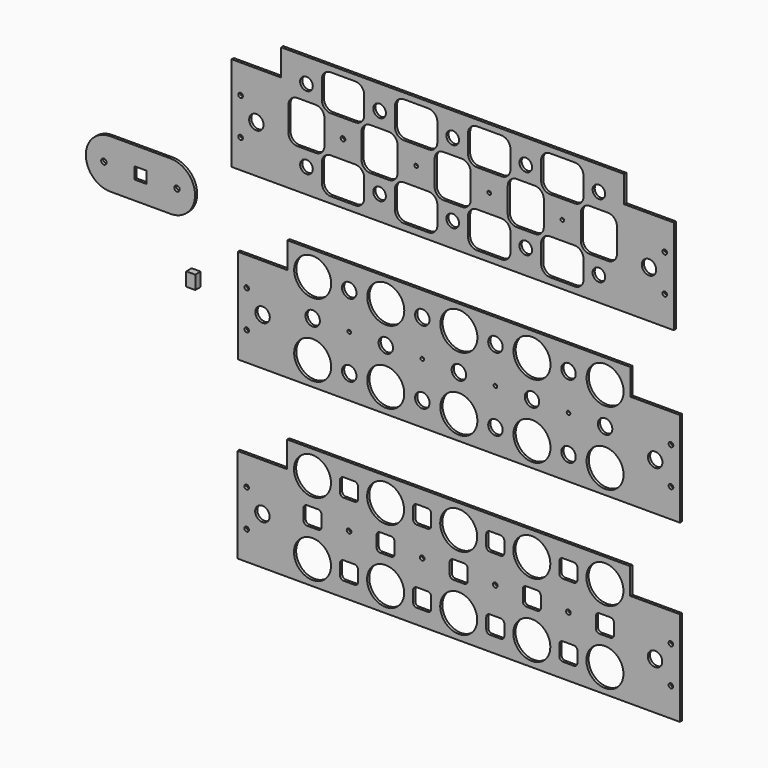
from build123d import *

# Parameters (mm, degrees)
F0_R     = 2.55
F0_R_2   = 8
F0_R_3   = 7
F0_R_4   = 2
F1_DEPTH = 3
F0_R_5   = 20.5
F0_W     = 20
F0_H     = 20
F2_DEPTH = 3
F0_R_6   = 3
F0_W_2   = 13
F0_H_2   = 13
F0_W_3   = 10
F0_H_3   = 15
F3_DEPTH = 4.5


# Not quite as in the source:
# - a feature names something its author has since deleted; it is built from what else it names


with BuildPart() as f1:
    # F0 (on Front) → F1 (new body)
    with BuildSketch(Plane.XZ):
        Polygon((-471.3846094865, 146.640773439), (-471.3846094865, 251.640773439), (-506.3846094865, 251.640773439), (-506.3846094865, 231.640773439), (-526.3846094865, 231.640773439), (-526.3846094865, 166.640773439), (-506.3846094865, 166.640773439), (-506.3846094865, 146.640773439), align=None)
        with Locations((-516.3846094865, 178.640773439)):
            Circle(F0_R, mode=Mode.SUBTRACT)
        with Locations((-498.8846094865, 199.140773439)):
            Circle(F0_R_2, mode=Mode.SUBTRACT)
        with Locations((-516.3846094865, 219.640773439)):
            Circle(F0_R, mode=Mode.SUBTRACT)
        Polygon((-56.3846094865, 251.640773439), (-91.3846094865, 251.640773439), (-91.3846094865, 146.640773439), (-56.3846094865, 146.640773439), (-56.3846094865, 166.640773439), (-36.3846094865, 166.640773439), (-36.3846094865, 231.640773439), (-56.3846094865, 231.640773439), align=None)
        with Locations((-46.3846094865, 178.640773439)):
            Circle(F0_R, mode=Mode.SUBTRACT)
        with Locations((-63.8846094865, 199.140773439)):
            Circle(F0_R_2, mode=Mode.SUBTRACT)
        with Locations((-46.3846094865, 219.640773439)):
            Circle(F0_R, mode=Mode.SUBTRACT)
        Polygon((-91.3846094865, 281.140773439), (-471.3846094865, 281.140773439), (-471.3846094865, 251.640773439), (-471.3846094865, 146.640773439), (-91.3846094865, 146.640773439), (-91.3846094865, 251.640773439), align=None)
        with Locations((-443.3846094865, 173.640773439)):
            Circle(F0_R_3, mode=Mode.SUBTRACT)
        with BuildLine():
            ThreePointArc((-433.399160381, 237.5500709947), (-426.3280925692, 234.6211388066), (-423.399160381, 227.5500709947))
            Line((-423.399160381, 227.5500709947), (-423.399160381, 200.5500709947))
            ThreePointArc((-423.399160381, 200.5500709947), (-426.3280925692, 193.4790031828), (-433.399160381, 190.5500709947))
            Line((-433.399160381, 190.5500709947), (-453.399160381, 190.5500709947))
            ThreePointArc((-453.399160381, 190.5500709947), (-460.4702281929, 193.4790031828), (-463.399160381, 200.5500709947))
            Line((-463.399160381, 200.5500709947), (-463.399160381, 227.5500709947))
            ThreePointArc((-463.399160381, 227.5500709947), (-460.4702281929, 234.6211388066), (-453.399160381, 237.5500709947))
            Line((-453.399160381, 237.5500709947), (-433.399160381, 237.5500709947))
        make_face(mode=Mode.SUBTRACT)
        with BuildLine():
            ThreePointArc((-379.3846094865, 163.640773439), (-382.3135416747, 156.5697056271), (-389.3846094865, 153.640773439))
            Line((-389.3846094865, 153.640773439), (-416.3846094865, 153.640773439))
            ThreePointArc((-416.3846094865, 153.640773439), (-423.4556772984, 156.5697056271), (-426.3846094865, 163.640773439))
            Line((-426.3846094865, 163.640773439), (-426.3846094865, 183.640773439))
            ThreePointArc((-426.3846094865, 183.640773439), (-423.4556772984, 190.7118412509), (-416.3846094865, 193.640773439))
            Line((-416.3846094865, 193.640773439), (-389.3846094865, 193.640773439))
            ThreePointArc((-389.3846094865, 193.640773439), (-382.3135416747, 190.7118412509), (-379.3846094865, 183.640773439))
            Line((-379.3846094865, 183.640773439), (-379.3846094865, 163.640773439))
        make_face(mode=Mode.SUBTRACT)
        with Locations((-362.3846094865, 173.640773439)):
            Circle(F0_R_3, mode=Mode.SUBTRACT)
        with Locations((-402.8846094865, 214.140773439)):
            Circle(F0_R, mode=Mode.SUBTRACT)
        with BuildLine():
            ThreePointArc((-352.399160381, 237.5500709947), (-345.3280925692, 234.6211388066), (-342.399160381, 227.5500709947))
            Line((-342.399160381, 227.5500709947), (-342.399160381, 200.5500709947))
            ThreePointArc((-342.399160381, 200.5500709947), (-345.3280925692, 193.4790031828), (-352.399160381, 190.5500709947))
            Line((-352.399160381, 190.5500709947), (-372.399160381, 190.5500709947))
            ThreePointArc((-372.399160381, 190.5500709947), (-379.4702281929, 193.4790031828), (-382.399160381, 200.5500709947))
            Line((-382.399160381, 200.5500709947), (-382.399160381, 227.5500709947))
            ThreePointArc((-382.399160381, 227.5500709947), (-379.4702281929, 234.6211388066), (-372.399160381, 237.5500709947))
            Line((-372.399160381, 237.5500709947), (-352.399160381, 237.5500709947))
        make_face(mode=Mode.SUBTRACT)
        with Locations((-443.3846094865, 254.640773439)):
            Circle(F0_R_3, mode=Mode.SUBTRACT)
        with BuildLine():
            ThreePointArc((-379.3846094865, 244.640773439), (-382.3135416747, 237.5697056271), (-389.3846094865, 234.640773439))
            Line((-389.3846094865, 234.640773439), (-416.3846094865, 234.640773439))
            ThreePointArc((-416.3846094865, 234.640773439), (-423.4556772984, 237.5697056271), (-426.3846094865, 244.640773439))
            Line((-426.3846094865, 244.640773439), (-426.3846094865, 264.640773439))
            ThreePointArc((-426.3846094865, 264.640773439), (-423.4556772984, 271.7118412509), (-416.3846094865, 274.640773439))
            Line((-416.3846094865, 274.640773439), (-389.3846094865, 274.640773439))
            ThreePointArc((-389.3846094865, 274.640773439), (-382.3135416747, 271.7118412509), (-379.3846094865, 264.640773439))
            Line((-379.3846094865, 264.640773439), (-379.3846094865, 244.640773439))
        make_face(mode=Mode.SUBTRACT)
        with Locations((-362.3846094865, 254.640773439)):
            Circle(F0_R_3, mode=Mode.SUBTRACT)
        with BuildLine():
            ThreePointArc((-298.3846094865, 163.640773439), (-301.3135416747, 156.5697056271), (-308.3846094865, 153.640773439))
            Line((-308.3846094865, 153.640773439), (-335.3846094865, 153.640773439))
            ThreePointArc((-335.3846094865, 153.640773439), (-342.4556772984, 156.5697056271), (-345.3846094865, 163.640773439))
            Line((-345.3846094865, 163.640773439), (-345.3846094865, 183.640773439))
            ThreePointArc((-345.3846094865, 183.640773439), (-342.4556772984, 190.7118412509), (-335.3846094865, 193.640773439))
            Line((-335.3846094865, 193.640773439), (-308.3846094865, 193.640773439))
            ThreePointArc((-308.3846094865, 193.640773439), (-301.3135416747, 190.7118412509), (-298.3846094865, 183.640773439))
            Line((-298.3846094865, 183.640773439), (-298.3846094865, 163.640773439))
        make_face(mode=Mode.SUBTRACT)
        with Locations((-281.3846094865, 173.640773439)):
            Circle(F0_R_3, mode=Mode.SUBTRACT)
        with Locations((-321.8846094865, 214.140773439)):
            Circle(F0_R_4, mode=Mode.SUBTRACT)
        with BuildLine():
            ThreePointArc((-271.399160381, 237.5500709947), (-264.3280925692, 234.6211388066), (-261.399160381, 227.5500709947))
            Line((-261.399160381, 227.5500709947), (-261.399160381, 200.5500709947))
            ThreePointArc((-261.399160381, 200.5500709947), (-264.3280925692, 193.4790031828), (-271.399160381, 190.5500709947))
            Line((-271.399160381, 190.5500709947), (-291.399160381, 190.5500709947))
            ThreePointArc((-291.399160381, 190.5500709947), (-298.4702281929, 193.4790031828), (-301.399160381, 200.5500709947))
            Line((-301.399160381, 200.5500709947), (-301.399160381, 227.5500709947))
            ThreePointArc((-301.399160381, 227.5500709947), (-298.4702281929, 234.6211388066), (-291.399160381, 237.5500709947))
            Line((-291.399160381, 237.5500709947), (-271.399160381, 237.5500709947))
        make_face(mode=Mode.SUBTRACT)
        with BuildLine():
            ThreePointArc((-217.3846094865, 163.640773439), (-220.3135416747, 156.5697056271), (-227.3846094865, 153.640773439))
            Line((-227.3846094865, 153.640773439), (-254.3846094865, 153.640773439))
            ThreePointArc((-254.3846094865, 153.640773439), (-261.4556772984, 156.5697056271), (-264.3846094865, 163.640773439))
            Line((-264.3846094865, 163.640773439), (-264.3846094865, 183.640773439))
            ThreePointArc((-264.3846094865, 183.640773439), (-261.4556772984, 190.7118412509), (-254.3846094865, 193.640773439))
            Line((-254.3846094865, 193.640773439), (-227.3846094865, 193.640773439))
            ThreePointArc((-227.3846094865, 193.640773439), (-220.3135416747, 190.7118412509), (-217.3846094865, 183.640773439))
            Line((-217.3846094865, 183.640773439), (-217.3846094865, 163.640773439))
        make_face(mode=Mode.SUBTRACT)
        with Locations((-200.3846094865, 173.640773439)):
            Circle(F0_R_3, mode=Mode.SUBTRACT)
        with Locations((-240.8846094865, 214.140773439)):
            Circle(F0_R_4, mode=Mode.SUBTRACT)
        with BuildLine():
            ThreePointArc((-190.399160381, 237.5500709947), (-183.3280925692, 234.6211388066), (-180.399160381, 227.5500709947))
            Line((-180.399160381, 227.5500709947), (-180.399160381, 200.5500709947))
            ThreePointArc((-180.399160381, 200.5500709947), (-183.3280925692, 193.4790031828), (-190.399160381, 190.5500709947))
            Line((-190.399160381, 190.5500709947), (-210.399160381, 190.5500709947))
            ThreePointArc((-210.399160381, 190.5500709947), (-217.4702281929, 193.4790031828), (-220.399160381, 200.5500709947))
            Line((-220.399160381, 200.5500709947), (-220.399160381, 227.5500709947))
            ThreePointArc((-220.399160381, 227.5500709947), (-217.4702281929, 234.6211388066), (-210.399160381, 237.5500709947))
            Line((-210.399160381, 237.5500709947), (-190.399160381, 237.5500709947))
        make_face(mode=Mode.SUBTRACT)
        with BuildLine():
            ThreePointArc((-298.3846094865, 244.640773439), (-301.3135416747, 237.5697056271), (-308.3846094865, 234.640773439))
            Line((-308.3846094865, 234.640773439), (-335.3846094865, 234.640773439))
            ThreePointArc((-335.3846094865, 234.640773439), (-342.4556772984, 237.5697056271), (-345.3846094865, 244.640773439))
            Line((-345.3846094865, 244.640773439), (-345.3846094865, 264.640773439))
            ThreePointArc((-345.3846094865, 264.640773439), (-342.4556772984, 271.7118412509), (-335.3846094865, 274.640773439))
            Line((-335.3846094865, 274.640773439), (-308.3846094865, 274.640773439))
            ThreePointArc((-308.3846094865, 274.640773439), (-301.3135416747, 271.7118412509), (-298.3846094865, 264.640773439))
            Line((-298.3846094865, 264.640773439), (-298.3846094865, 244.640773439))
        make_face(mode=Mode.SUBTRACT)
        with Locations((-281.3846094865, 254.640773439)):
            Circle(F0_R_3, mode=Mode.SUBTRACT)
        with BuildLine():
            ThreePointArc((-217.3846094865, 244.640773439), (-220.3135416747, 237.5697056271), (-227.3846094865, 234.640773439))
            Line((-227.3846094865, 234.640773439), (-254.3846094865, 234.640773439))
            ThreePointArc((-254.3846094865, 234.640773439), (-261.4556772984, 237.5697056271), (-264.3846094865, 244.640773439))
            Line((-264.3846094865, 244.640773439), (-264.3846094865, 264.640773439))
            ThreePointArc((-264.3846094865, 264.640773439), (-261.4556772984, 271.7118412509), (-254.3846094865, 274.640773439))
            Line((-254.3846094865, 274.640773439), (-227.3846094865, 274.640773439))
            ThreePointArc((-227.3846094865, 274.640773439), (-220.3135416747, 271.7118412509), (-217.3846094865, 264.640773439))
            Line((-217.3846094865, 264.640773439), (-217.3846094865, 244.640773439))
        make_face(mode=Mode.SUBTRACT)
        with Locations((-200.3846094865, 254.640773439)):
            Circle(F0_R_3, mode=Mode.SUBTRACT)
        with BuildLine():
            ThreePointArc((-136.3846094865, 163.640773439), (-139.3135416747, 156.5697056271), (-146.3846094865, 153.640773439))
            Line((-146.3846094865, 153.640773439), (-173.3846094865, 153.640773439))
            ThreePointArc((-173.3846094865, 153.640773439), (-180.4556772984, 156.5697056271), (-183.3846094865, 163.640773439))
            Line((-183.3846094865, 163.640773439), (-183.3846094865, 183.640773439))
            ThreePointArc((-183.3846094865, 183.640773439), (-180.4556772984, 190.7118412509), (-173.3846094865, 193.640773439))
            Line((-173.3846094865, 193.640773439), (-146.3846094865, 193.640773439))
            ThreePointArc((-146.3846094865, 193.640773439), (-139.3135416747, 190.7118412509), (-136.3846094865, 183.640773439))
            Line((-136.3846094865, 183.640773439), (-136.3846094865, 163.640773439))
        make_face(mode=Mode.SUBTRACT)
        with Locations((-119.3846094865, 173.640773439)):
            Circle(F0_R_3, mode=Mode.SUBTRACT)
        with Locations((-159.8846094865, 214.140773439)):
            Circle(F0_R_4, mode=Mode.SUBTRACT)
        with BuildLine():
            ThreePointArc((-109.399160381, 237.5500709947), (-102.3280925692, 234.6211388066), (-99.399160381, 227.5500709947))
            Line((-99.399160381, 227.5500709947), (-99.399160381, 200.5500709947))
            ThreePointArc((-99.399160381, 200.5500709947), (-102.3280925692, 193.4790031828), (-109.399160381, 190.5500709947))
            Line((-109.399160381, 190.5500709947), (-129.399160381, 190.5500709947))
            ThreePointArc((-129.399160381, 190.5500709947), (-136.4702281929, 193.4790031828), (-139.399160381, 200.5500709947))
            Line((-139.399160381, 200.5500709947), (-139.399160381, 227.5500709947))
            ThreePointArc((-139.399160381, 227.5500709947), (-136.4702281929, 234.6211388066), (-129.399160381, 237.5500709947))
            Line((-129.399160381, 237.5500709947), (-109.399160381, 237.5500709947))
        make_face(mode=Mode.SUBTRACT)
        with BuildLine():
            ThreePointArc((-136.3846094865, 244.640773439), (-139.3135416747, 237.5697056271), (-146.3846094865, 234.640773439))
            Line((-146.3846094865, 234.640773439), (-173.3846094865, 234.640773439))
            ThreePointArc((-173.3846094865, 234.640773439), (-180.4556772984, 237.5697056271), (-183.3846094865, 244.640773439))
            Line((-183.3846094865, 244.640773439), (-183.3846094865, 264.640773439))
            ThreePointArc((-183.3846094865, 264.640773439), (-180.4556772984, 271.7118412509), (-173.3846094865, 274.640773439))
            Line((-173.3846094865, 274.640773439), (-146.3846094865, 274.640773439))
            ThreePointArc((-146.3846094865, 274.640773439), (-139.3135416747, 271.7118412509), (-136.3846094865, 264.640773439))
            Line((-136.3846094865, 264.640773439), (-136.3846094865, 244.640773439))
        make_face(mode=Mode.SUBTRACT)
        with Locations((-119.3846094865, 254.640773439)):
            Circle(F0_R_3, mode=Mode.SUBTRACT)
    extrude(amount=F1_DEPTH)


with BuildPart() as f1b:
    # F0 (on Front) → F1, piece 2 (new body)
    with BuildSketch(Plane.XZ):
        Polygon((-84.5069469546, 95.13103152), (-464.5069469546, 95.13103152), (-464.5069469546, 66.13103152), (-464.5069469546, -38.86896848), (-84.5069469546, -38.86896848), (-84.5069469546, 66.13103152), align=None)
        with Locations((-436.5069469546, -12.36896848)):
            Circle(F0_R_5, mode=Mode.SUBTRACT)
        with BuildLine():
            ThreePointArc((-388.0069469546, -12.36896848), (-396.0069469546, -20.36896848), (-404.0069469546, -12.36896848))
            ThreePointArc((-404.0069469546, -12.36896848), (-396.0069469546, -4.36896848), (-388.0069469546, -12.36896848))
        make_face(mode=Mode.SUBTRACT)
        with BuildLine():
            ThreePointArc((-335.0069469546, -12.36896848), (-355.5069469546, -32.86896848), (-376.0069469546, -12.36896848))
            ThreePointArc((-376.0069469546, -12.36896848), (-355.5069469546, 8.13103152), (-335.0069469546, -12.36896848))
        make_face(mode=Mode.SUBTRACT)
        with Locations((-315.0069469546, -12.36896848)):
            Circle(F0_R_2, mode=Mode.SUBTRACT)
        with Locations((-274.5069469546, -12.36896848)):
            Circle(F0_R_5, mode=Mode.SUBTRACT)
        with Locations((-234.0069469546, -12.36896848)):
            Circle(F0_R_2, mode=Mode.SUBTRACT)
        with Locations((-193.5069469546, -12.36896848)):
            Circle(F0_R_5, mode=Mode.SUBTRACT)
        with Locations((-153.0069469546, -12.36896848)):
            Circle(F0_R_2, mode=Mode.SUBTRACT)
        with Locations((-112.5069469546, -12.36896848)):
            Circle(F0_R_5, mode=Mode.SUBTRACT)
        with Locations((-436.5069469546, 28.13103152)):
            Circle(F0_R_2, mode=Mode.SUBTRACT)
        with Locations((-396.0069469546, 28.13103152)):
            Circle(F0_R_4, mode=Mode.SUBTRACT)
        with Locations((-436.5069469546, 68.63103152)):
            Circle(F0_R_5, mode=Mode.SUBTRACT)
        with Locations((-396.0069469546, 68.63103152)):
            Circle(F0_R_2, mode=Mode.SUBTRACT)
        with Locations((-355.5069469546, 28.13103152)):
            Circle(F0_R_2, mode=Mode.SUBTRACT)
        with Locations((-315.0069469546, 28.13103152)):
            Circle(F0_R_4, mode=Mode.SUBTRACT)
        with Locations((-355.5069469546, 68.63103152)):
            Circle(F0_R_5, mode=Mode.SUBTRACT)
        with Locations((-315.0069469546, 68.63103152)):
            Circle(F0_R_2, mode=Mode.SUBTRACT)
        with Locations((-274.5069469546, 28.13103152)):
            Circle(F0_R_2, mode=Mode.SUBTRACT)
        with Locations((-234.0069469546, 28.13103152)):
            Circle(F0_R_4, mode=Mode.SUBTRACT)
        with Locations((-274.5069469546, 68.63103152)):
            Circle(F0_R_5, mode=Mode.SUBTRACT)
        with Locations((-234.0069469546, 68.63103152)):
            Circle(F0_R_2, mode=Mode.SUBTRACT)
        with Locations((-193.5069469546, 28.13103152)):
            Circle(F0_R_2, mode=Mode.SUBTRACT)
        with Locations((-153.0069469546, 28.13103152)):
            Circle(F0_R_4, mode=Mode.SUBTRACT)
        with Locations((-112.5069469546, 28.13103152)):
            Circle(F0_R_2, mode=Mode.SUBTRACT)
        with Locations((-193.5069469546, 68.63103152)):
            Circle(F0_R_5, mode=Mode.SUBTRACT)
        with Locations((-153.0069469546, 68.63103152)):
            Circle(F0_R_2, mode=Mode.SUBTRACT)
        with Locations((-112.5069469546, 68.63103152)):
            Circle(F0_R_5, mode=Mode.SUBTRACT)
        Polygon((-464.5069469546, -38.86896848), (-464.5069469546, 66.13103152), (-499.5069469546, 66.13103152), (-499.5069469546, 46.13103152), (-519.5069469546, 46.13103152), (-519.5069469546, -18.86896848), (-499.5069469546, -18.86896848), (-499.5069469546, -38.86896848), align=None)
        with Locations((-509.5069469546, -6.86896848)):
            Circle(F0_R, mode=Mode.SUBTRACT)
        with Locations((-492.0069469546, 13.63103152)):
            Circle(F0_R_2, mode=Mode.SUBTRACT)
        with Locations((-509.5069469546, 34.13103152)):
            Circle(F0_R, mode=Mode.SUBTRACT)
        Polygon((-49.5069469546, 66.13103152), (-84.5069469546, 66.13103152), (-84.5069469546, -38.86896848), (-49.5069469546, -38.86896848), (-49.5069469546, -18.86896848), (-29.5069469546, -18.86896848), (-29.5069469546, 46.13103152), (-49.5069469546, 46.13103152), align=None)
        with Locations((-39.5069469546, -6.86896848)):
            Circle(F0_R, mode=Mode.SUBTRACT)
        with Locations((-57.0069469546, 13.63103152)):
            Circle(F0_R_2, mode=Mode.SUBTRACT)
        with Locations((-39.5069469546, 34.13103152)):
            Circle(F0_R, mode=Mode.SUBTRACT)
    extrude(amount=F1_DEPTH)


with BuildPart() as f1c:
    # F0 (on Front) → F1, piece 3 (new body)
    with BuildSketch(Plane.XZ):
        Polygon((-49.6968317032, -128.2062721252), (-84.6968317032, -128.2062721252), (-84.6968317032, -233.2062721252), (-49.6968317032, -233.2062721252), (-49.6968317032, -213.2062721252), (-29.6968317032, -213.2062721252), (-29.6968317032, -148.2062721252), (-49.6968317032, -148.2062721252), align=None)
        with Locations((-39.6968317032, -201.2062721252)):
            Circle(F0_R, mode=Mode.SUBTRACT)
        with Locations((-57.1968317032, -180.7062721252)):
            Circle(F0_R_2, mode=Mode.SUBTRACT)
        with Locations((-39.6968317032, -160.2062721252)):
            Circle(F0_R, mode=Mode.SUBTRACT)
        Polygon((-84.6968317032, -99.2062721252), (-464.6968317032, -99.2062721252), (-464.6968317032, -128.2062721252), (-464.6968317032, -233.2062721252), (-84.6968317032, -233.2062721252), (-84.6968317032, -128.2062721252), align=None)
        with Locations((-436.6968317032, -206.7062721252)):
            Circle(F0_R_5, mode=Mode.SUBTRACT)
        with BuildLine():
            Line((-406.1968317032, -212.7062721252), (-406.1968317032, -206.7062721252))
            Line((-406.1968317032, -206.7062721252), (-406.1968317032, -200.7062721252))
            ThreePointArc((-406.1968317032, -200.7062721252), (-405.0252588279, -197.8778450005), (-402.1968317032, -196.7062721252))
            Line((-402.1968317032, -196.7062721252), (-390.1968317032, -196.7062721252))
            ThreePointArc((-390.1968317032, -196.7062721252), (-387.3684045784, -197.8778450005), (-386.1968317032, -200.7062721252))
            Line((-386.1968317032, -200.7062721252), (-386.1968317032, -206.7062721252))
            Line((-386.1968317032, -206.7062721252), (-386.1968317032, -212.7062721252))
            ThreePointArc((-386.1968317032, -212.7062721252), (-387.3684045784, -215.53469925), (-390.1968317032, -216.7062721252))
            Line((-390.1968317032, -216.7062721252), (-402.1968317032, -216.7062721252))
            ThreePointArc((-402.1968317032, -216.7062721252), (-405.0252588279, -215.53469925), (-406.1968317032, -212.7062721252))
        make_face(mode=Mode.SUBTRACT)
        with BuildLine():
            ThreePointArc((-426.6968317032, -172.2062721252), (-427.8684045784, -175.03469925), (-430.6968317032, -176.2062721252))
            Line((-430.6968317032, -176.2062721252), (-442.6968317032, -176.2062721252))
            ThreePointArc((-442.6968317032, -176.2062721252), (-445.5252588279, -175.03469925), (-446.6968317032, -172.2062721252))
            Line((-446.6968317032, -172.2062721252), (-446.6968317032, -160.2062721252))
            ThreePointArc((-446.6968317032, -160.2062721252), (-445.5252588279, -157.3778450005), (-442.6968317032, -156.2062721252))
            Line((-442.6968317032, -156.2062721252), (-430.6968317032, -156.2062721252))
            ThreePointArc((-430.6968317032, -156.2062721252), (-427.8684045784, -157.3778450005), (-426.6968317032, -160.2062721252))
            Line((-426.6968317032, -160.2062721252), (-426.6968317032, -172.2062721252))
        make_face(mode=Mode.SUBTRACT)
        with Locations((-396.1968317032, -166.2062721252)):
            Circle(F0_R, mode=Mode.SUBTRACT)
        with Locations((-436.6968317032, -125.7062721252)):
            Circle(F0_R_5, mode=Mode.SUBTRACT)
        with BuildLine():
            ThreePointArc((-386.1968317032, -131.7062721252), (-387.3684045784, -134.53469925), (-390.1968317032, -135.7062721252))
            Line((-390.1968317032, -135.7062721252), (-402.1968317032, -135.7062721252))
            ThreePointArc((-402.1968317032, -135.7062721252), (-405.0252588279, -134.53469925), (-406.1968317032, -131.7062721252))
            Line((-406.1968317032, -131.7062721252), (-406.1968317032, -119.7062721252))
            ThreePointArc((-406.1968317032, -119.7062721252), (-405.0252588279, -116.8778450005), (-402.1968317032, -115.7062721252))
            Line((-402.1968317032, -115.7062721252), (-390.1968317032, -115.7062721252))
            ThreePointArc((-390.1968317032, -115.7062721252), (-387.3684045784, -116.8778450005), (-386.1968317032, -119.7062721252))
            Line((-386.1968317032, -119.7062721252), (-386.1968317032, -131.7062721252))
        make_face(mode=Mode.SUBTRACT)
        with BuildLine():
            ThreePointArc((-335.1968317032, -206.7062721252), (-355.6968317032, -227.2062721252), (-376.1968317032, -206.7062721252))
            ThreePointArc((-376.1968317032, -206.7062721252), (-355.6968317032, -186.2062721252), (-335.1968317032, -206.7062721252))
        make_face(mode=Mode.SUBTRACT)
        with BuildLine():
            ThreePointArc((-305.1968317032, -212.7062721252), (-306.3684045784, -215.53469925), (-309.1968317032, -216.7062721252))
            Line((-309.1968317032, -216.7062721252), (-321.1968317032, -216.7062721252))
            ThreePointArc((-321.1968317032, -216.7062721252), (-324.0252588279, -215.53469925), (-325.1968317032, -212.7062721252))
            Line((-325.1968317032, -212.7062721252), (-325.1968317032, -200.7062721252))
            ThreePointArc((-325.1968317032, -200.7062721252), (-324.0252588279, -197.8778450005), (-321.1968317032, -196.7062721252))
            Line((-321.1968317032, -196.7062721252), (-309.1968317032, -196.7062721252))
            ThreePointArc((-309.1968317032, -196.7062721252), (-306.3684045784, -197.8778450005), (-305.1968317032, -200.7062721252))
            Line((-305.1968317032, -200.7062721252), (-305.1968317032, -212.7062721252))
        make_face(mode=Mode.SUBTRACT)
        with Locations((-274.6968317032, -206.7062721252)):
            Circle(F0_R_5, mode=Mode.SUBTRACT)
        with BuildLine():
            ThreePointArc((-224.1968317032, -212.7062721252), (-225.3684045784, -215.53469925), (-228.1968317032, -216.7062721252))
            Line((-228.1968317032, -216.7062721252), (-240.1968317032, -216.7062721252))
            ThreePointArc((-240.1968317032, -216.7062721252), (-243.0252588279, -215.53469925), (-244.1968317032, -212.7062721252))
            Line((-244.1968317032, -212.7062721252), (-244.1968317032, -200.7062721252))
            ThreePointArc((-244.1968317032, -200.7062721252), (-243.0252588279, -197.8778450005), (-240.1968317032, -196.7062721252))
            Line((-240.1968317032, -196.7062721252), (-228.1968317032, -196.7062721252))
            ThreePointArc((-228.1968317032, -196.7062721252), (-225.3684045784, -197.8778450005), (-224.1968317032, -200.7062721252))
            Line((-224.1968317032, -200.7062721252), (-224.1968317032, -212.7062721252))
        make_face(mode=Mode.SUBTRACT)
        with BuildLine():
            ThreePointArc((-361.6968317032, -176.2062721252), (-364.5252588279, -175.03469925), (-365.6968317032, -172.2062721252))
            Line((-365.6968317032, -172.2062721252), (-365.6968317032, -160.2062721252))
            ThreePointArc((-365.6968317032, -160.2062721252), (-364.5252588279, -157.3778450005), (-361.6968317032, -156.2062721252))
            Line((-361.6968317032, -156.2062721252), (-349.6968317032, -156.2062721252))
            ThreePointArc((-349.6968317032, -156.2062721252), (-346.8684045784, -157.3778450005), (-345.6968317032, -160.2062721252))
            Line((-345.6968317032, -160.2062721252), (-345.6968317032, -172.2062721252))
            ThreePointArc((-345.6968317032, -172.2062721252), (-346.8684045784, -175.03469925), (-349.6968317032, -176.2062721252))
            Line((-349.6968317032, -176.2062721252), (-361.6968317032, -176.2062721252))
        make_face(mode=Mode.SUBTRACT)
        with Locations((-315.1968317032, -166.2062721252)):
            Circle(F0_R, mode=Mode.SUBTRACT)
        with Locations((-355.6968317032, -125.7062721252)):
            Circle(F0_R_5, mode=Mode.SUBTRACT)
        with BuildLine():
            ThreePointArc((-305.1968317032, -131.7062721252), (-306.3684045784, -134.53469925), (-309.1968317032, -135.7062721252))
            Line((-309.1968317032, -135.7062721252), (-321.1968317032, -135.7062721252))
            ThreePointArc((-321.1968317032, -135.7062721252), (-324.0252588279, -134.53469925), (-325.1968317032, -131.7062721252))
            Line((-325.1968317032, -131.7062721252), (-325.1968317032, -119.7062721252))
            ThreePointArc((-325.1968317032, -119.7062721252), (-324.0252588279, -116.8778450005), (-321.1968317032, -115.7062721252))
            Line((-321.1968317032, -115.7062721252), (-309.1968317032, -115.7062721252))
            ThreePointArc((-309.1968317032, -115.7062721252), (-306.3684045784, -116.8778450005), (-305.1968317032, -119.7062721252))
            Line((-305.1968317032, -119.7062721252), (-305.1968317032, -131.7062721252))
        make_face(mode=Mode.SUBTRACT)
        with BuildLine():
            ThreePointArc((-280.6968317032, -176.2062721252), (-283.5252588279, -175.03469925), (-284.6968317032, -172.2062721252))
            Line((-284.6968317032, -172.2062721252), (-284.6968317032, -160.2062721252))
            ThreePointArc((-284.6968317032, -160.2062721252), (-283.5252588279, -157.3778450005), (-280.6968317032, -156.2062721252))
            Line((-280.6968317032, -156.2062721252), (-268.6968317032, -156.2062721252))
            ThreePointArc((-268.6968317032, -156.2062721252), (-265.8684045784, -157.3778450005), (-264.6968317032, -160.2062721252))
            Line((-264.6968317032, -160.2062721252), (-264.6968317032, -172.2062721252))
            ThreePointArc((-264.6968317032, -172.2062721252), (-265.8684045784, -175.03469925), (-268.6968317032, -176.2062721252))
            Line((-268.6968317032, -176.2062721252), (-280.6968317032, -176.2062721252))
        make_face(mode=Mode.SUBTRACT)
        with Locations((-234.1968317032, -166.2062721252)):
            Circle(F0_R, mode=Mode.SUBTRACT)
        with Locations((-274.6968317032, -125.7062721252)):
            Circle(F0_R_5, mode=Mode.SUBTRACT)
        with BuildLine():
            ThreePointArc((-224.1968317032, -131.7062721252), (-225.3684045784, -134.53469925), (-228.1968317032, -135.7062721252))
            Line((-228.1968317032, -135.7062721252), (-240.1968317032, -135.7062721252))
            ThreePointArc((-240.1968317032, -135.7062721252), (-243.0252588279, -134.53469925), (-244.1968317032, -131.7062721252))
            Line((-244.1968317032, -131.7062721252), (-244.1968317032, -119.7062721252))
            ThreePointArc((-244.1968317032, -119.7062721252), (-243.0252588279, -116.8778450005), (-240.1968317032, -115.7062721252))
            Line((-240.1968317032, -115.7062721252), (-228.1968317032, -115.7062721252))
            ThreePointArc((-228.1968317032, -115.7062721252), (-225.3684045784, -116.8778450005), (-224.1968317032, -119.7062721252))
            Line((-224.1968317032, -119.7062721252), (-224.1968317032, -131.7062721252))
        make_face(mode=Mode.SUBTRACT)
        with Locations((-193.6968317032, -206.7062721252)):
            Circle(F0_R_5, mode=Mode.SUBTRACT)
        with BuildLine():
            ThreePointArc((-143.1968317032, -212.7062721252), (-144.3684045784, -215.53469925), (-147.1968317032, -216.7062721252))
            Line((-147.1968317032, -216.7062721252), (-159.1968317032, -216.7062721252))
            ThreePointArc((-159.1968317032, -216.7062721252), (-162.0252588279, -215.53469925), (-163.1968317032, -212.7062721252))
            Line((-163.1968317032, -212.7062721252), (-163.1968317032, -200.7062721252))
            ThreePointArc((-163.1968317032, -200.7062721252), (-162.0252588279, -197.8778450005), (-159.1968317032, -196.7062721252))
            Line((-159.1968317032, -196.7062721252), (-147.1968317032, -196.7062721252))
            ThreePointArc((-147.1968317032, -196.7062721252), (-144.3684045784, -197.8778450005), (-143.1968317032, -200.7062721252))
            Line((-143.1968317032, -200.7062721252), (-143.1968317032, -212.7062721252))
        make_face(mode=Mode.SUBTRACT)
        with Locations((-112.6968317032, -206.7062721252)):
            Circle(F0_R_5, mode=Mode.SUBTRACT)
        with BuildLine():
            ThreePointArc((-199.6968317032, -176.2062721252), (-202.5252588279, -175.03469925), (-203.6968317032, -172.2062721252))
            Line((-203.6968317032, -172.2062721252), (-203.6968317032, -160.2062721252))
            ThreePointArc((-203.6968317032, -160.2062721252), (-202.5252588279, -157.3778450005), (-199.6968317032, -156.2062721252))
            Line((-199.6968317032, -156.2062721252), (-187.6968317032, -156.2062721252))
            ThreePointArc((-187.6968317032, -156.2062721252), (-184.8684045784, -157.3778450005), (-183.6968317032, -160.2062721252))
            Line((-183.6968317032, -160.2062721252), (-183.6968317032, -172.2062721252))
            ThreePointArc((-183.6968317032, -172.2062721252), (-184.8684045784, -175.03469925), (-187.6968317032, -176.2062721252))
            Line((-187.6968317032, -176.2062721252), (-199.6968317032, -176.2062721252))
        make_face(mode=Mode.SUBTRACT)
        with Locations((-153.1968317032, -166.2062721252)):
            Circle(F0_R, mode=Mode.SUBTRACT)
        with BuildLine():
            ThreePointArc((-118.6968317032, -176.2062721252), (-121.5252588279, -175.03469925), (-122.6968317032, -172.2062721252))
            Line((-122.6968317032, -172.2062721252), (-122.6968317032, -160.2062721252))
            ThreePointArc((-122.6968317032, -160.2062721252), (-121.5252588279, -157.3778450005), (-118.6968317032, -156.2062721252))
            Line((-118.6968317032, -156.2062721252), (-106.6968317032, -156.2062721252))
            ThreePointArc((-106.6968317032, -156.2062721252), (-103.8684045784, -157.3778450005), (-102.6968317032, -160.2062721252))
            Line((-102.6968317032, -160.2062721252), (-102.6968317032, -172.2062721252))
            ThreePointArc((-102.6968317032, -172.2062721252), (-103.8684045784, -175.03469925), (-106.6968317032, -176.2062721252))
            Line((-106.6968317032, -176.2062721252), (-118.6968317032, -176.2062721252))
        make_face(mode=Mode.SUBTRACT)
        with Locations((-193.6968317032, -125.7062721252)):
            Circle(F0_R_5, mode=Mode.SUBTRACT)
        with BuildLine():
            ThreePointArc((-143.1968317032, -131.7062721252), (-144.3684045784, -134.53469925), (-147.1968317032, -135.7062721252))
            Line((-147.1968317032, -135.7062721252), (-159.1968317032, -135.7062721252))
            ThreePointArc((-159.1968317032, -135.7062721252), (-162.0252588279, -134.53469925), (-163.1968317032, -131.7062721252))
            Line((-163.1968317032, -131.7062721252), (-163.1968317032, -119.7062721252))
            ThreePointArc((-163.1968317032, -119.7062721252), (-162.0252588279, -116.8778450005), (-159.1968317032, -115.7062721252))
            Line((-159.1968317032, -115.7062721252), (-147.1968317032, -115.7062721252))
            ThreePointArc((-147.1968317032, -115.7062721252), (-144.3684045784, -116.8778450005), (-143.1968317032, -119.7062721252))
            Line((-143.1968317032, -119.7062721252), (-143.1968317032, -131.7062721252))
        make_face(mode=Mode.SUBTRACT)
        with Locations((-112.6968317032, -125.7062721252)):
            Circle(F0_R_5, mode=Mode.SUBTRACT)
        Polygon((-464.6968317032, -233.2062721252), (-464.6968317032, -128.2062721252), (-499.6968317032, -128.2062721252), (-499.6968317032, -148.2062721252), (-519.6968317032, -148.2062721252), (-519.6968317032, -213.2062721252), (-499.6968317032, -213.2062721252), (-499.6968317032, -233.2062721252), align=None)
        with Locations((-509.6968317032, -201.2062721252)):
            Circle(F0_R, mode=Mode.SUBTRACT)
        with Locations((-492.1968317032, -180.7062721252)):
            Circle(F0_R_2, mode=Mode.SUBTRACT)
        with Locations((-509.6968317032, -160.2062721252)):
            Circle(F0_R, mode=Mode.SUBTRACT)
    extrude(amount=F1_DEPTH)


with BuildPart() as f2:
    # F0 (on Front) → F2 (new body)
    with BuildSketch(Plane.XZ):
        Polygon((-91.3846094865, 281.140773439), (-471.3846094865, 281.140773439), (-471.3846094865, 251.640773439), (-471.3846094865, 146.640773439), (-91.3846094865, 146.640773439), (-91.3846094865, 251.640773439), align=None)
        with Locations((-443.3846094865, 173.640773439)):
            Circle(F0_R_3, mode=Mode.SUBTRACT)
        with BuildLine():
            ThreePointArc((-433.399160381, 237.5500709947), (-426.3280925692, 234.6211388066), (-423.399160381, 227.5500709947))
            Line((-423.399160381, 227.5500709947), (-423.399160381, 200.5500709947))
            ThreePointArc((-423.399160381, 200.5500709947), (-426.3280925692, 193.4790031828), (-433.399160381, 190.5500709947))
            Line((-433.399160381, 190.5500709947), (-453.399160381, 190.5500709947))
            ThreePointArc((-453.399160381, 190.5500709947), (-460.4702281929, 193.4790031828), (-463.399160381, 200.5500709947))
            Line((-463.399160381, 200.5500709947), (-463.399160381, 227.5500709947))
            ThreePointArc((-463.399160381, 227.5500709947), (-460.4702281929, 234.6211388066), (-453.399160381, 237.5500709947))
            Line((-453.399160381, 237.5500709947), (-433.399160381, 237.5500709947))
        make_face(mode=Mode.SUBTRACT)
        with BuildLine():
            ThreePointArc((-379.3846094865, 163.640773439), (-382.3135416747, 156.5697056271), (-389.3846094865, 153.640773439))
            Line((-389.3846094865, 153.640773439), (-416.3846094865, 153.640773439))
            ThreePointArc((-416.3846094865, 153.640773439), (-423.4556772984, 156.5697056271), (-426.3846094865, 163.640773439))
            Line((-426.3846094865, 163.640773439), (-426.3846094865, 183.640773439))
            ThreePointArc((-426.3846094865, 183.640773439), (-423.4556772984, 190.7118412509), (-416.3846094865, 193.640773439))
            Line((-416.3846094865, 193.640773439), (-389.3846094865, 193.640773439))
            ThreePointArc((-389.3846094865, 193.640773439), (-382.3135416747, 190.7118412509), (-379.3846094865, 183.640773439))
            Line((-379.3846094865, 183.640773439), (-379.3846094865, 163.640773439))
        make_face(mode=Mode.SUBTRACT)
        with Locations((-362.3846094865, 173.640773439)):
            Circle(F0_R_3, mode=Mode.SUBTRACT)
        with Locations((-402.8846094865, 214.140773439)):
            Circle(F0_R, mode=Mode.SUBTRACT)
        with BuildLine():
            ThreePointArc((-352.399160381, 237.5500709947), (-345.3280925692, 234.6211388066), (-342.399160381, 227.5500709947))
            Line((-342.399160381, 227.5500709947), (-342.399160381, 200.5500709947))
            ThreePointArc((-342.399160381, 200.5500709947), (-345.3280925692, 193.4790031828), (-352.399160381, 190.5500709947))
            Line((-352.399160381, 190.5500709947), (-372.399160381, 190.5500709947))
            ThreePointArc((-372.399160381, 190.5500709947), (-379.4702281929, 193.4790031828), (-382.399160381, 200.5500709947))
            Line((-382.399160381, 200.5500709947), (-382.399160381, 227.5500709947))
            ThreePointArc((-382.399160381, 227.5500709947), (-379.4702281929, 234.6211388066), (-372.399160381, 237.5500709947))
            Line((-372.399160381, 237.5500709947), (-352.399160381, 237.5500709947))
        make_face(mode=Mode.SUBTRACT)
        with Locations((-443.3846094865, 254.640773439)):
            Circle(F0_R_3, mode=Mode.SUBTRACT)
        with BuildLine():
            ThreePointArc((-379.3846094865, 244.640773439), (-382.3135416747, 237.5697056271), (-389.3846094865, 234.640773439))
            Line((-389.3846094865, 234.640773439), (-416.3846094865, 234.640773439))
            ThreePointArc((-416.3846094865, 234.640773439), (-423.4556772984, 237.5697056271), (-426.3846094865, 244.640773439))
            Line((-426.3846094865, 244.640773439), (-426.3846094865, 264.640773439))
            ThreePointArc((-426.3846094865, 264.640773439), (-423.4556772984, 271.7118412509), (-416.3846094865, 274.640773439))
            Line((-416.3846094865, 274.640773439), (-389.3846094865, 274.640773439))
            ThreePointArc((-389.3846094865, 274.640773439), (-382.3135416747, 271.7118412509), (-379.3846094865, 264.640773439))
            Line((-379.3846094865, 264.640773439), (-379.3846094865, 244.640773439))
        make_face(mode=Mode.SUBTRACT)
        with Locations((-362.3846094865, 254.640773439)):
            Circle(F0_R_3, mode=Mode.SUBTRACT)
        with BuildLine():
            ThreePointArc((-298.3846094865, 163.640773439), (-301.3135416747, 156.5697056271), (-308.3846094865, 153.640773439))
            Line((-308.3846094865, 153.640773439), (-335.3846094865, 153.640773439))
            ThreePointArc((-335.3846094865, 153.640773439), (-342.4556772984, 156.5697056271), (-345.3846094865, 163.640773439))
            Line((-345.3846094865, 163.640773439), (-345.3846094865, 183.640773439))
            ThreePointArc((-345.3846094865, 183.640773439), (-342.4556772984, 190.7118412509), (-335.3846094865, 193.640773439))
            Line((-335.3846094865, 193.640773439), (-308.3846094865, 193.640773439))
            ThreePointArc((-308.3846094865, 193.640773439), (-301.3135416747, 190.7118412509), (-298.3846094865, 183.640773439))
            Line((-298.3846094865, 183.640773439), (-298.3846094865, 163.640773439))
        make_face(mode=Mode.SUBTRACT)
        with Locations((-281.3846094865, 173.640773439)):
            Circle(F0_R_3, mode=Mode.SUBTRACT)
        with Locations((-321.8846094865, 214.140773439)):
            Circle(F0_R_4, mode=Mode.SUBTRACT)
        with BuildLine():
            ThreePointArc((-271.399160381, 237.5500709947), (-264.3280925692, 234.6211388066), (-261.399160381, 227.5500709947))
            Line((-261.399160381, 227.5500709947), (-261.399160381, 200.5500709947))
            ThreePointArc((-261.399160381, 200.5500709947), (-264.3280925692, 193.4790031828), (-271.399160381, 190.5500709947))
            Line((-271.399160381, 190.5500709947), (-291.399160381, 190.5500709947))
            ThreePointArc((-291.399160381, 190.5500709947), (-298.4702281929, 193.4790031828), (-301.399160381, 200.5500709947))
            Line((-301.399160381, 200.5500709947), (-301.399160381, 227.5500709947))
            ThreePointArc((-301.399160381, 227.5500709947), (-298.4702281929, 234.6211388066), (-291.399160381, 237.5500709947))
            Line((-291.399160381, 237.5500709947), (-271.399160381, 237.5500709947))
        make_face(mode=Mode.SUBTRACT)
        with BuildLine():
            ThreePointArc((-217.3846094865, 163.640773439), (-220.3135416747, 156.5697056271), (-227.3846094865, 153.640773439))
            Line((-227.3846094865, 153.640773439), (-254.3846094865, 153.640773439))
            ThreePointArc((-254.3846094865, 153.640773439), (-261.4556772984, 156.5697056271), (-264.3846094865, 163.640773439))
            Line((-264.3846094865, 163.640773439), (-264.3846094865, 183.640773439))
            ThreePointArc((-264.3846094865, 183.640773439), (-261.4556772984, 190.7118412509), (-254.3846094865, 193.640773439))
            Line((-254.3846094865, 193.640773439), (-227.3846094865, 193.640773439))
            ThreePointArc((-227.3846094865, 193.640773439), (-220.3135416747, 190.7118412509), (-217.3846094865, 183.640773439))
            Line((-217.3846094865, 183.640773439), (-217.3846094865, 163.640773439))
        make_face(mode=Mode.SUBTRACT)
        with Locations((-200.3846094865, 173.640773439)):
            Circle(F0_R_3, mode=Mode.SUBTRACT)
        with Locations((-240.8846094865, 214.140773439)):
            Circle(F0_R_4, mode=Mode.SUBTRACT)
        with BuildLine():
            ThreePointArc((-190.399160381, 237.5500709947), (-183.3280925692, 234.6211388066), (-180.399160381, 227.5500709947))
            Line((-180.399160381, 227.5500709947), (-180.399160381, 200.5500709947))
            ThreePointArc((-180.399160381, 200.5500709947), (-183.3280925692, 193.4790031828), (-190.399160381, 190.5500709947))
            Line((-190.399160381, 190.5500709947), (-210.399160381, 190.5500709947))
            ThreePointArc((-210.399160381, 190.5500709947), (-217.4702281929, 193.4790031828), (-220.399160381, 200.5500709947))
            Line((-220.399160381, 200.5500709947), (-220.399160381, 227.5500709947))
            ThreePointArc((-220.399160381, 227.5500709947), (-217.4702281929, 234.6211388066), (-210.399160381, 237.5500709947))
            Line((-210.399160381, 237.5500709947), (-190.399160381, 237.5500709947))
        make_face(mode=Mode.SUBTRACT)
        with BuildLine():
            ThreePointArc((-298.3846094865, 244.640773439), (-301.3135416747, 237.5697056271), (-308.3846094865, 234.640773439))
            Line((-308.3846094865, 234.640773439), (-335.3846094865, 234.640773439))
            ThreePointArc((-335.3846094865, 234.640773439), (-342.4556772984, 237.5697056271), (-345.3846094865, 244.640773439))
            Line((-345.3846094865, 244.640773439), (-345.3846094865, 264.640773439))
            ThreePointArc((-345.3846094865, 264.640773439), (-342.4556772984, 271.7118412509), (-335.3846094865, 274.640773439))
            Line((-335.3846094865, 274.640773439), (-308.3846094865, 274.640773439))
            ThreePointArc((-308.3846094865, 274.640773439), (-301.3135416747, 271.7118412509), (-298.3846094865, 264.640773439))
            Line((-298.3846094865, 264.640773439), (-298.3846094865, 244.640773439))
        make_face(mode=Mode.SUBTRACT)
        with Locations((-281.3846094865, 254.640773439)):
            Circle(F0_R_3, mode=Mode.SUBTRACT)
        with BuildLine():
            ThreePointArc((-217.3846094865, 244.640773439), (-220.3135416747, 237.5697056271), (-227.3846094865, 234.640773439))
            Line((-227.3846094865, 234.640773439), (-254.3846094865, 234.640773439))
            ThreePointArc((-254.3846094865, 234.640773439), (-261.4556772984, 237.5697056271), (-264.3846094865, 244.640773439))
            Line((-264.3846094865, 244.640773439), (-264.3846094865, 264.640773439))
            ThreePointArc((-264.3846094865, 264.640773439), (-261.4556772984, 271.7118412509), (-254.3846094865, 274.640773439))
            Line((-254.3846094865, 274.640773439), (-227.3846094865, 274.640773439))
            ThreePointArc((-227.3846094865, 274.640773439), (-220.3135416747, 271.7118412509), (-217.3846094865, 264.640773439))
            Line((-217.3846094865, 264.640773439), (-217.3846094865, 244.640773439))
        make_face(mode=Mode.SUBTRACT)
        with Locations((-200.3846094865, 254.640773439)):
            Circle(F0_R_3, mode=Mode.SUBTRACT)
        with BuildLine():
            ThreePointArc((-136.3846094865, 163.640773439), (-139.3135416747, 156.5697056271), (-146.3846094865, 153.640773439))
            Line((-146.3846094865, 153.640773439), (-173.3846094865, 153.640773439))
            ThreePointArc((-173.3846094865, 153.640773439), (-180.4556772984, 156.5697056271), (-183.3846094865, 163.640773439))
            Line((-183.3846094865, 163.640773439), (-183.3846094865, 183.640773439))
            ThreePointArc((-183.3846094865, 183.640773439), (-180.4556772984, 190.7118412509), (-173.3846094865, 193.640773439))
            Line((-173.3846094865, 193.640773439), (-146.3846094865, 193.640773439))
            ThreePointArc((-146.3846094865, 193.640773439), (-139.3135416747, 190.7118412509), (-136.3846094865, 183.640773439))
            Line((-136.3846094865, 183.640773439), (-136.3846094865, 163.640773439))
        make_face(mode=Mode.SUBTRACT)
        with Locations((-119.3846094865, 173.640773439)):
            Circle(F0_R_3, mode=Mode.SUBTRACT)
        with Locations((-159.8846094865, 214.140773439)):
            Circle(F0_R_4, mode=Mode.SUBTRACT)
        with BuildLine():
            ThreePointArc((-109.399160381, 237.5500709947), (-102.3280925692, 234.6211388066), (-99.399160381, 227.5500709947))
            Line((-99.399160381, 227.5500709947), (-99.399160381, 200.5500709947))
            ThreePointArc((-99.399160381, 200.5500709947), (-102.3280925692, 193.4790031828), (-109.399160381, 190.5500709947))
            Line((-109.399160381, 190.5500709947), (-129.399160381, 190.5500709947))
            ThreePointArc((-129.399160381, 190.5500709947), (-136.4702281929, 193.4790031828), (-139.399160381, 200.5500709947))
            Line((-139.399160381, 200.5500709947), (-139.399160381, 227.5500709947))
            ThreePointArc((-139.399160381, 227.5500709947), (-136.4702281929, 234.6211388066), (-129.399160381, 237.5500709947))
            Line((-129.399160381, 237.5500709947), (-109.399160381, 237.5500709947))
        make_face(mode=Mode.SUBTRACT)
        with BuildLine():
            ThreePointArc((-136.3846094865, 244.640773439), (-139.3135416747, 237.5697056271), (-146.3846094865, 234.640773439))
            Line((-146.3846094865, 234.640773439), (-173.3846094865, 234.640773439))
            ThreePointArc((-173.3846094865, 234.640773439), (-180.4556772984, 237.5697056271), (-183.3846094865, 244.640773439))
            Line((-183.3846094865, 244.640773439), (-183.3846094865, 264.640773439))
            ThreePointArc((-183.3846094865, 264.640773439), (-180.4556772984, 271.7118412509), (-173.3846094865, 274.640773439))
            Line((-173.3846094865, 274.640773439), (-146.3846094865, 274.640773439))
            ThreePointArc((-146.3846094865, 274.640773439), (-139.3135416747, 271.7118412509), (-136.3846094865, 264.640773439))
            Line((-136.3846094865, 264.640773439), (-136.3846094865, 244.640773439))
        make_face(mode=Mode.SUBTRACT)
        with Locations((-119.3846094865, 254.640773439)):
            Circle(F0_R_3, mode=Mode.SUBTRACT)
        Polygon((-471.3846094865, 146.640773439), (-471.3846094865, 251.640773439), (-506.3846094865, 251.640773439), (-506.3846094865, 231.640773439), (-526.3846094865, 231.640773439), (-526.3846094865, 166.640773439), (-506.3846094865, 166.640773439), (-506.3846094865, 146.640773439), align=None)
        with Locations((-516.3846094865, 178.640773439)):
            Circle(F0_R, mode=Mode.SUBTRACT)
        with Locations((-498.8846094865, 199.140773439)):
            Circle(F0_R_2, mode=Mode.SUBTRACT)
        with Locations((-516.3846094865, 219.640773439)):
            Circle(F0_R, mode=Mode.SUBTRACT)
        Polygon((-56.3846094865, 251.640773439), (-91.3846094865, 251.640773439), (-91.3846094865, 146.640773439), (-56.3846094865, 146.640773439), (-56.3846094865, 166.640773439), (-36.3846094865, 166.640773439), (-36.3846094865, 231.640773439), (-56.3846094865, 231.640773439), align=None)
        with Locations((-46.3846094865, 178.640773439)):
            Circle(F0_R, mode=Mode.SUBTRACT)
        with Locations((-63.8846094865, 199.140773439)):
            Circle(F0_R_2, mode=Mode.SUBTRACT)
        with Locations((-46.3846094865, 219.640773439)):
            Circle(F0_R, mode=Mode.SUBTRACT)
        with Locations((-516.3846094865, 241.640773439)):
            Rectangle(F0_W, F0_H)
        with Locations((-46.3846094865, 241.640773439)):
            Rectangle(F0_W, F0_H)
        with Locations((-516.3846094865, 156.640773439)):
            Rectangle(F0_W, F0_H)
        with Locations((-46.3846094865, 156.640773439)):
            Rectangle(F0_W, F0_H)
    extrude(amount=F2_DEPTH)


with BuildPart() as f2b:
    # F0 (on Front) → F2, piece 2 (new body)
    with BuildSketch(Plane.XZ):
        Polygon((-84.5069469546, 95.13103152), (-464.5069469546, 95.13103152), (-464.5069469546, 66.13103152), (-464.5069469546, -38.86896848), (-84.5069469546, -38.86896848), (-84.5069469546, 66.13103152), align=None)
        with Locations((-436.5069469546, -12.36896848)):
            Circle(F0_R_5, mode=Mode.SUBTRACT)
        with BuildLine():
            ThreePointArc((-388.0069469546, -12.36896848), (-396.0069469546, -20.36896848), (-404.0069469546, -12.36896848))
            ThreePointArc((-404.0069469546, -12.36896848), (-396.0069469546, -4.36896848), (-388.0069469546, -12.36896848))
        make_face(mode=Mode.SUBTRACT)
        with BuildLine():
            ThreePointArc((-335.0069469546, -12.36896848), (-355.5069469546, -32.86896848), (-376.0069469546, -12.36896848))
            ThreePointArc((-376.0069469546, -12.36896848), (-355.5069469546, 8.13103152), (-335.0069469546, -12.36896848))
        make_face(mode=Mode.SUBTRACT)
        with Locations((-315.0069469546, -12.36896848)):
            Circle(F0_R_2, mode=Mode.SUBTRACT)
        with Locations((-274.5069469546, -12.36896848)):
            Circle(F0_R_5, mode=Mode.SUBTRACT)
        with Locations((-234.0069469546, -12.36896848)):
            Circle(F0_R_2, mode=Mode.SUBTRACT)
        with Locations((-193.5069469546, -12.36896848)):
            Circle(F0_R_5, mode=Mode.SUBTRACT)
        with Locations((-153.0069469546, -12.36896848)):
            Circle(F0_R_2, mode=Mode.SUBTRACT)
        with Locations((-112.5069469546, -12.36896848)):
            Circle(F0_R_5, mode=Mode.SUBTRACT)
        with Locations((-436.5069469546, 28.13103152)):
            Circle(F0_R_2, mode=Mode.SUBTRACT)
        with Locations((-396.0069469546, 28.13103152)):
            Circle(F0_R_4, mode=Mode.SUBTRACT)
        with Locations((-436.5069469546, 68.63103152)):
            Circle(F0_R_5, mode=Mode.SUBTRACT)
        with Locations((-396.0069469546, 68.63103152)):
            Circle(F0_R_2, mode=Mode.SUBTRACT)
        with Locations((-355.5069469546, 28.13103152)):
            Circle(F0_R_2, mode=Mode.SUBTRACT)
        with Locations((-315.0069469546, 28.13103152)):
            Circle(F0_R_4, mode=Mode.SUBTRACT)
        with Locations((-355.5069469546, 68.63103152)):
            Circle(F0_R_5, mode=Mode.SUBTRACT)
        with Locations((-315.0069469546, 68.63103152)):
            Circle(F0_R_2, mode=Mode.SUBTRACT)
        with Locations((-274.5069469546, 28.13103152)):
            Circle(F0_R_2, mode=Mode.SUBTRACT)
        with Locations((-234.0069469546, 28.13103152)):
            Circle(F0_R_4, mode=Mode.SUBTRACT)
        with Locations((-274.5069469546, 68.63103152)):
            Circle(F0_R_5, mode=Mode.SUBTRACT)
        with Locations((-234.0069469546, 68.63103152)):
            Circle(F0_R_2, mode=Mode.SUBTRACT)
        with Locations((-193.5069469546, 28.13103152)):
            Circle(F0_R_2, mode=Mode.SUBTRACT)
        with Locations((-153.0069469546, 28.13103152)):
            Circle(F0_R_4, mode=Mode.SUBTRACT)
        with Locations((-112.5069469546, 28.13103152)):
            Circle(F0_R_2, mode=Mode.SUBTRACT)
        with Locations((-193.5069469546, 68.63103152)):
            Circle(F0_R_5, mode=Mode.SUBTRACT)
        with Locations((-153.0069469546, 68.63103152)):
            Circle(F0_R_2, mode=Mode.SUBTRACT)
        with Locations((-112.5069469546, 68.63103152)):
            Circle(F0_R_5, mode=Mode.SUBTRACT)
        Polygon((-464.5069469546, -38.86896848), (-464.5069469546, 66.13103152), (-499.5069469546, 66.13103152), (-499.5069469546, 46.13103152), (-519.5069469546, 46.13103152), (-519.5069469546, -18.86896848), (-499.5069469546, -18.86896848), (-499.5069469546, -38.86896848), align=None)
        with Locations((-509.5069469546, -6.86896848)):
            Circle(F0_R, mode=Mode.SUBTRACT)
        with Locations((-492.0069469546, 13.63103152)):
            Circle(F0_R_2, mode=Mode.SUBTRACT)
        with Locations((-509.5069469546, 34.13103152)):
            Circle(F0_R, mode=Mode.SUBTRACT)
        Polygon((-49.5069469546, 66.13103152), (-84.5069469546, 66.13103152), (-84.5069469546, -38.86896848), (-49.5069469546, -38.86896848), (-49.5069469546, -18.86896848), (-29.5069469546, -18.86896848), (-29.5069469546, 46.13103152), (-49.5069469546, 46.13103152), align=None)
        with Locations((-39.5069469546, -6.86896848)):
            Circle(F0_R, mode=Mode.SUBTRACT)
        with Locations((-57.0069469546, 13.63103152)):
            Circle(F0_R_2, mode=Mode.SUBTRACT)
        with Locations((-39.5069469546, 34.13103152)):
            Circle(F0_R, mode=Mode.SUBTRACT)
        with Locations((-509.5069469546, 56.13103152)):
            Rectangle(F0_W, F0_H)
        with Locations((-39.5069469546, 56.13103152)):
            Rectangle(F0_W, F0_H)
        with Locations((-509.5069469546, -28.86896848)):
            Rectangle(F0_W, F0_H)
        with Locations((-39.5069469546, -28.86896848)):
            Rectangle(F0_W, F0_H)
    extrude(amount=F2_DEPTH)


with BuildPart() as f2c:
    # F0 (on Front) → F2, piece 3 (new body)
    with BuildSketch(Plane.XZ):
        Polygon((-84.6968317032, -99.2062721252), (-464.6968317032, -99.2062721252), (-464.6968317032, -128.2062721252), (-464.6968317032, -233.2062721252), (-84.6968317032, -233.2062721252), (-84.6968317032, -128.2062721252), align=None)
        with Locations((-436.6968317032, -206.7062721252)):
            Circle(F0_R_5, mode=Mode.SUBTRACT)
        with BuildLine():
            Line((-406.1968317032, -212.7062721252), (-406.1968317032, -206.7062721252))
            Line((-406.1968317032, -206.7062721252), (-406.1968317032, -200.7062721252))
            ThreePointArc((-406.1968317032, -200.7062721252), (-405.0252588279, -197.8778450005), (-402.1968317032, -196.7062721252))
            Line((-402.1968317032, -196.7062721252), (-390.1968317032, -196.7062721252))
            ThreePointArc((-390.1968317032, -196.7062721252), (-387.3684045784, -197.8778450005), (-386.1968317032, -200.7062721252))
            Line((-386.1968317032, -200.7062721252), (-386.1968317032, -206.7062721252))
            Line((-386.1968317032, -206.7062721252), (-386.1968317032, -212.7062721252))
            ThreePointArc((-386.1968317032, -212.7062721252), (-387.3684045784, -215.53469925), (-390.1968317032, -216.7062721252))
            Line((-390.1968317032, -216.7062721252), (-402.1968317032, -216.7062721252))
            ThreePointArc((-402.1968317032, -216.7062721252), (-405.0252588279, -215.53469925), (-406.1968317032, -212.7062721252))
        make_face(mode=Mode.SUBTRACT)
        with BuildLine():
            ThreePointArc((-426.6968317032, -172.2062721252), (-427.8684045784, -175.03469925), (-430.6968317032, -176.2062721252))
            Line((-430.6968317032, -176.2062721252), (-442.6968317032, -176.2062721252))
            ThreePointArc((-442.6968317032, -176.2062721252), (-445.5252588279, -175.03469925), (-446.6968317032, -172.2062721252))
            Line((-446.6968317032, -172.2062721252), (-446.6968317032, -160.2062721252))
            ThreePointArc((-446.6968317032, -160.2062721252), (-445.5252588279, -157.3778450005), (-442.6968317032, -156.2062721252))
            Line((-442.6968317032, -156.2062721252), (-430.6968317032, -156.2062721252))
            ThreePointArc((-430.6968317032, -156.2062721252), (-427.8684045784, -157.3778450005), (-426.6968317032, -160.2062721252))
            Line((-426.6968317032, -160.2062721252), (-426.6968317032, -172.2062721252))
        make_face(mode=Mode.SUBTRACT)
        with Locations((-396.1968317032, -166.2062721252)):
            Circle(F0_R, mode=Mode.SUBTRACT)
        with Locations((-436.6968317032, -125.7062721252)):
            Circle(F0_R_5, mode=Mode.SUBTRACT)
        with BuildLine():
            ThreePointArc((-386.1968317032, -131.7062721252), (-387.3684045784, -134.53469925), (-390.1968317032, -135.7062721252))
            Line((-390.1968317032, -135.7062721252), (-402.1968317032, -135.7062721252))
            ThreePointArc((-402.1968317032, -135.7062721252), (-405.0252588279, -134.53469925), (-406.1968317032, -131.7062721252))
            Line((-406.1968317032, -131.7062721252), (-406.1968317032, -119.7062721252))
            ThreePointArc((-406.1968317032, -119.7062721252), (-405.0252588279, -116.8778450005), (-402.1968317032, -115.7062721252))
            Line((-402.1968317032, -115.7062721252), (-390.1968317032, -115.7062721252))
            ThreePointArc((-390.1968317032, -115.7062721252), (-387.3684045784, -116.8778450005), (-386.1968317032, -119.7062721252))
            Line((-386.1968317032, -119.7062721252), (-386.1968317032, -131.7062721252))
        make_face(mode=Mode.SUBTRACT)
        with BuildLine():
            ThreePointArc((-335.1968317032, -206.7062721252), (-355.6968317032, -227.2062721252), (-376.1968317032, -206.7062721252))
            ThreePointArc((-376.1968317032, -206.7062721252), (-355.6968317032, -186.2062721252), (-335.1968317032, -206.7062721252))
        make_face(mode=Mode.SUBTRACT)
        with BuildLine():
            ThreePointArc((-305.1968317032, -212.7062721252), (-306.3684045784, -215.53469925), (-309.1968317032, -216.7062721252))
            Line((-309.1968317032, -216.7062721252), (-321.1968317032, -216.7062721252))
            ThreePointArc((-321.1968317032, -216.7062721252), (-324.0252588279, -215.53469925), (-325.1968317032, -212.7062721252))
            Line((-325.1968317032, -212.7062721252), (-325.1968317032, -200.7062721252))
            ThreePointArc((-325.1968317032, -200.7062721252), (-324.0252588279, -197.8778450005), (-321.1968317032, -196.7062721252))
            Line((-321.1968317032, -196.7062721252), (-309.1968317032, -196.7062721252))
            ThreePointArc((-309.1968317032, -196.7062721252), (-306.3684045784, -197.8778450005), (-305.1968317032, -200.7062721252))
            Line((-305.1968317032, -200.7062721252), (-305.1968317032, -212.7062721252))
        make_face(mode=Mode.SUBTRACT)
        with Locations((-274.6968317032, -206.7062721252)):
            Circle(F0_R_5, mode=Mode.SUBTRACT)
        with BuildLine():
            ThreePointArc((-224.1968317032, -212.7062721252), (-225.3684045784, -215.53469925), (-228.1968317032, -216.7062721252))
            Line((-228.1968317032, -216.7062721252), (-240.1968317032, -216.7062721252))
            ThreePointArc((-240.1968317032, -216.7062721252), (-243.0252588279, -215.53469925), (-244.1968317032, -212.7062721252))
            Line((-244.1968317032, -212.7062721252), (-244.1968317032, -200.7062721252))
            ThreePointArc((-244.1968317032, -200.7062721252), (-243.0252588279, -197.8778450005), (-240.1968317032, -196.7062721252))
            Line((-240.1968317032, -196.7062721252), (-228.1968317032, -196.7062721252))
            ThreePointArc((-228.1968317032, -196.7062721252), (-225.3684045784, -197.8778450005), (-224.1968317032, -200.7062721252))
            Line((-224.1968317032, -200.7062721252), (-224.1968317032, -212.7062721252))
        make_face(mode=Mode.SUBTRACT)
        with BuildLine():
            ThreePointArc((-361.6968317032, -176.2062721252), (-364.5252588279, -175.03469925), (-365.6968317032, -172.2062721252))
            Line((-365.6968317032, -172.2062721252), (-365.6968317032, -160.2062721252))
            ThreePointArc((-365.6968317032, -160.2062721252), (-364.5252588279, -157.3778450005), (-361.6968317032, -156.2062721252))
            Line((-361.6968317032, -156.2062721252), (-349.6968317032, -156.2062721252))
            ThreePointArc((-349.6968317032, -156.2062721252), (-346.8684045784, -157.3778450005), (-345.6968317032, -160.2062721252))
            Line((-345.6968317032, -160.2062721252), (-345.6968317032, -172.2062721252))
            ThreePointArc((-345.6968317032, -172.2062721252), (-346.8684045784, -175.03469925), (-349.6968317032, -176.2062721252))
            Line((-349.6968317032, -176.2062721252), (-361.6968317032, -176.2062721252))
        make_face(mode=Mode.SUBTRACT)
        with Locations((-315.1968317032, -166.2062721252)):
            Circle(F0_R, mode=Mode.SUBTRACT)
        with Locations((-355.6968317032, -125.7062721252)):
            Circle(F0_R_5, mode=Mode.SUBTRACT)
        with BuildLine():
            ThreePointArc((-305.1968317032, -131.7062721252), (-306.3684045784, -134.53469925), (-309.1968317032, -135.7062721252))
            Line((-309.1968317032, -135.7062721252), (-321.1968317032, -135.7062721252))
            ThreePointArc((-321.1968317032, -135.7062721252), (-324.0252588279, -134.53469925), (-325.1968317032, -131.7062721252))
            Line((-325.1968317032, -131.7062721252), (-325.1968317032, -119.7062721252))
            ThreePointArc((-325.1968317032, -119.7062721252), (-324.0252588279, -116.8778450005), (-321.1968317032, -115.7062721252))
            Line((-321.1968317032, -115.7062721252), (-309.1968317032, -115.7062721252))
            ThreePointArc((-309.1968317032, -115.7062721252), (-306.3684045784, -116.8778450005), (-305.1968317032, -119.7062721252))
            Line((-305.1968317032, -119.7062721252), (-305.1968317032, -131.7062721252))
        make_face(mode=Mode.SUBTRACT)
        with BuildLine():
            ThreePointArc((-280.6968317032, -176.2062721252), (-283.5252588279, -175.03469925), (-284.6968317032, -172.2062721252))
            Line((-284.6968317032, -172.2062721252), (-284.6968317032, -160.2062721252))
            ThreePointArc((-284.6968317032, -160.2062721252), (-283.5252588279, -157.3778450005), (-280.6968317032, -156.2062721252))
            Line((-280.6968317032, -156.2062721252), (-268.6968317032, -156.2062721252))
            ThreePointArc((-268.6968317032, -156.2062721252), (-265.8684045784, -157.3778450005), (-264.6968317032, -160.2062721252))
            Line((-264.6968317032, -160.2062721252), (-264.6968317032, -172.2062721252))
            ThreePointArc((-264.6968317032, -172.2062721252), (-265.8684045784, -175.03469925), (-268.6968317032, -176.2062721252))
            Line((-268.6968317032, -176.2062721252), (-280.6968317032, -176.2062721252))
        make_face(mode=Mode.SUBTRACT)
        with Locations((-234.1968317032, -166.2062721252)):
            Circle(F0_R, mode=Mode.SUBTRACT)
        with Locations((-274.6968317032, -125.7062721252)):
            Circle(F0_R_5, mode=Mode.SUBTRACT)
        with BuildLine():
            ThreePointArc((-224.1968317032, -131.7062721252), (-225.3684045784, -134.53469925), (-228.1968317032, -135.7062721252))
            Line((-228.1968317032, -135.7062721252), (-240.1968317032, -135.7062721252))
            ThreePointArc((-240.1968317032, -135.7062721252), (-243.0252588279, -134.53469925), (-244.1968317032, -131.7062721252))
            Line((-244.1968317032, -131.7062721252), (-244.1968317032, -119.7062721252))
            ThreePointArc((-244.1968317032, -119.7062721252), (-243.0252588279, -116.8778450005), (-240.1968317032, -115.7062721252))
            Line((-240.1968317032, -115.7062721252), (-228.1968317032, -115.7062721252))
            ThreePointArc((-228.1968317032, -115.7062721252), (-225.3684045784, -116.8778450005), (-224.1968317032, -119.7062721252))
            Line((-224.1968317032, -119.7062721252), (-224.1968317032, -131.7062721252))
        make_face(mode=Mode.SUBTRACT)
        with Locations((-193.6968317032, -206.7062721252)):
            Circle(F0_R_5, mode=Mode.SUBTRACT)
        with BuildLine():
            ThreePointArc((-143.1968317032, -212.7062721252), (-144.3684045784, -215.53469925), (-147.1968317032, -216.7062721252))
            Line((-147.1968317032, -216.7062721252), (-159.1968317032, -216.7062721252))
            ThreePointArc((-159.1968317032, -216.7062721252), (-162.0252588279, -215.53469925), (-163.1968317032, -212.7062721252))
            Line((-163.1968317032, -212.7062721252), (-163.1968317032, -200.7062721252))
            ThreePointArc((-163.1968317032, -200.7062721252), (-162.0252588279, -197.8778450005), (-159.1968317032, -196.7062721252))
            Line((-159.1968317032, -196.7062721252), (-147.1968317032, -196.7062721252))
            ThreePointArc((-147.1968317032, -196.7062721252), (-144.3684045784, -197.8778450005), (-143.1968317032, -200.7062721252))
            Line((-143.1968317032, -200.7062721252), (-143.1968317032, -212.7062721252))
        make_face(mode=Mode.SUBTRACT)
        with Locations((-112.6968317032, -206.7062721252)):
            Circle(F0_R_5, mode=Mode.SUBTRACT)
        with BuildLine():
            ThreePointArc((-199.6968317032, -176.2062721252), (-202.5252588279, -175.03469925), (-203.6968317032, -172.2062721252))
            Line((-203.6968317032, -172.2062721252), (-203.6968317032, -160.2062721252))
            ThreePointArc((-203.6968317032, -160.2062721252), (-202.5252588279, -157.3778450005), (-199.6968317032, -156.2062721252))
            Line((-199.6968317032, -156.2062721252), (-187.6968317032, -156.2062721252))
            ThreePointArc((-187.6968317032, -156.2062721252), (-184.8684045784, -157.3778450005), (-183.6968317032, -160.2062721252))
            Line((-183.6968317032, -160.2062721252), (-183.6968317032, -172.2062721252))
            ThreePointArc((-183.6968317032, -172.2062721252), (-184.8684045784, -175.03469925), (-187.6968317032, -176.2062721252))
            Line((-187.6968317032, -176.2062721252), (-199.6968317032, -176.2062721252))
        make_face(mode=Mode.SUBTRACT)
        with Locations((-153.1968317032, -166.2062721252)):
            Circle(F0_R, mode=Mode.SUBTRACT)
        with BuildLine():
            ThreePointArc((-118.6968317032, -176.2062721252), (-121.5252588279, -175.03469925), (-122.6968317032, -172.2062721252))
            Line((-122.6968317032, -172.2062721252), (-122.6968317032, -160.2062721252))
            ThreePointArc((-122.6968317032, -160.2062721252), (-121.5252588279, -157.3778450005), (-118.6968317032, -156.2062721252))
            Line((-118.6968317032, -156.2062721252), (-106.6968317032, -156.2062721252))
            ThreePointArc((-106.6968317032, -156.2062721252), (-103.8684045784, -157.3778450005), (-102.6968317032, -160.2062721252))
            Line((-102.6968317032, -160.2062721252), (-102.6968317032, -172.2062721252))
            ThreePointArc((-102.6968317032, -172.2062721252), (-103.8684045784, -175.03469925), (-106.6968317032, -176.2062721252))
            Line((-106.6968317032, -176.2062721252), (-118.6968317032, -176.2062721252))
        make_face(mode=Mode.SUBTRACT)
        with Locations((-193.6968317032, -125.7062721252)):
            Circle(F0_R_5, mode=Mode.SUBTRACT)
        with BuildLine():
            ThreePointArc((-143.1968317032, -131.7062721252), (-144.3684045784, -134.53469925), (-147.1968317032, -135.7062721252))
            Line((-147.1968317032, -135.7062721252), (-159.1968317032, -135.7062721252))
            ThreePointArc((-159.1968317032, -135.7062721252), (-162.0252588279, -134.53469925), (-163.1968317032, -131.7062721252))
            Line((-163.1968317032, -131.7062721252), (-163.1968317032, -119.7062721252))
            ThreePointArc((-163.1968317032, -119.7062721252), (-162.0252588279, -116.8778450005), (-159.1968317032, -115.7062721252))
            Line((-159.1968317032, -115.7062721252), (-147.1968317032, -115.7062721252))
            ThreePointArc((-147.1968317032, -115.7062721252), (-144.3684045784, -116.8778450005), (-143.1968317032, -119.7062721252))
            Line((-143.1968317032, -119.7062721252), (-143.1968317032, -131.7062721252))
        make_face(mode=Mode.SUBTRACT)
        with Locations((-112.6968317032, -125.7062721252)):
            Circle(F0_R_5, mode=Mode.SUBTRACT)
        Polygon((-464.6968317032, -233.2062721252), (-464.6968317032, -128.2062721252), (-499.6968317032, -128.2062721252), (-499.6968317032, -148.2062721252), (-519.6968317032, -148.2062721252), (-519.6968317032, -213.2062721252), (-499.6968317032, -213.2062721252), (-499.6968317032, -233.2062721252), align=None)
        with Locations((-509.6968317032, -201.2062721252)):
            Circle(F0_R, mode=Mode.SUBTRACT)
        with Locations((-492.1968317032, -180.7062721252)):
            Circle(F0_R_2, mode=Mode.SUBTRACT)
        with Locations((-509.6968317032, -160.2062721252)):
            Circle(F0_R, mode=Mode.SUBTRACT)
        Polygon((-49.6968317032, -128.2062721252), (-84.6968317032, -128.2062721252), (-84.6968317032, -233.2062721252), (-49.6968317032, -233.2062721252), (-49.6968317032, -213.2062721252), (-29.6968317032, -213.2062721252), (-29.6968317032, -148.2062721252), (-49.6968317032, -148.2062721252), align=None)
        with Locations((-39.6968317032, -201.2062721252)):
            Circle(F0_R, mode=Mode.SUBTRACT)
        with Locations((-57.1968317032, -180.7062721252)):
            Circle(F0_R_2, mode=Mode.SUBTRACT)
        with Locations((-39.6968317032, -160.2062721252)):
            Circle(F0_R, mode=Mode.SUBTRACT)
        with Locations((-509.6968317032, -138.2062721252)):
            Rectangle(F0_W, F0_H)
        with Locations((-39.6968317032, -138.2062721252)):
            Rectangle(F0_W, F0_H)
        with Locations((-509.6968317032, -223.2062721252)):
            Rectangle(F0_W, F0_H)
        with Locations((-39.6968317032, -223.2062721252)):
            Rectangle(F0_W, F0_H)
    extrude(amount=F2_DEPTH)


with BuildPart() as f2d:
    # F0 (on Front) → F2, piece 4 (new body)
    with BuildSketch(Plane.XZ):
        with BuildLine():
            Line((-660.832508564, 78.8227568865), (-593.832508564, 78.8227568865))
            ThreePointArc((-593.832508564, 78.8227568865), (-574.740625472, 86.7308737944), (-566.832508564, 105.8227568865))
            ThreePointArc((-566.832508564, 105.8227568865), (-574.740625472, 124.9146399785), (-593.832508564, 132.8227568865))
            Line((-593.832508564, 132.8227568865), (-660.832508564, 132.8227568865))
            ThreePointArc((-660.832508564, 132.8227568865), (-679.924391656, 124.9146399785), (-687.832508564, 105.8227568865))
            ThreePointArc((-687.832508564, 105.8227568865), (-679.924391656, 86.7308737944), (-660.832508564, 78.8227568865))
        make_face()
        with Locations((-667.832508564, 105.8227568865)):
            Circle(F0_R_6, mode=Mode.SUBTRACT)
        with Locations((-627.332508564, 105.8227568865)):
            Rectangle(F0_W_2, F0_H_2, mode=Mode.SUBTRACT)
        with Locations((-586.832508564, 105.8227568865)):
            Circle(F0_R_6, mode=Mode.SUBTRACT)
    extrude(amount=F2_DEPTH)


with BuildPart() as f2e:
    # F0 (on Front) → F2, piece 5 (new body)
    with BuildSketch(Plane.XZ):
        with Locations((-567.9844617844, 23.9318255335)):
            Rectangle(F0_W_3, F0_H_3)
    extrude(amount=F2_DEPTH)

    # F3 (add): a face of the model
    f3_faces = [f2e.faces().sort_by_distance(p)[0] for p in [
        (-567.9844617844, -3, 23.9318255335),
    ]]
    extrude(f3_faces, amount=F3_DEPTH)


solid = Compound([f1.part, f1b.part, f1c.part, f2.part, f2b.part, f2c.part, f2d.part, f2e.part])
